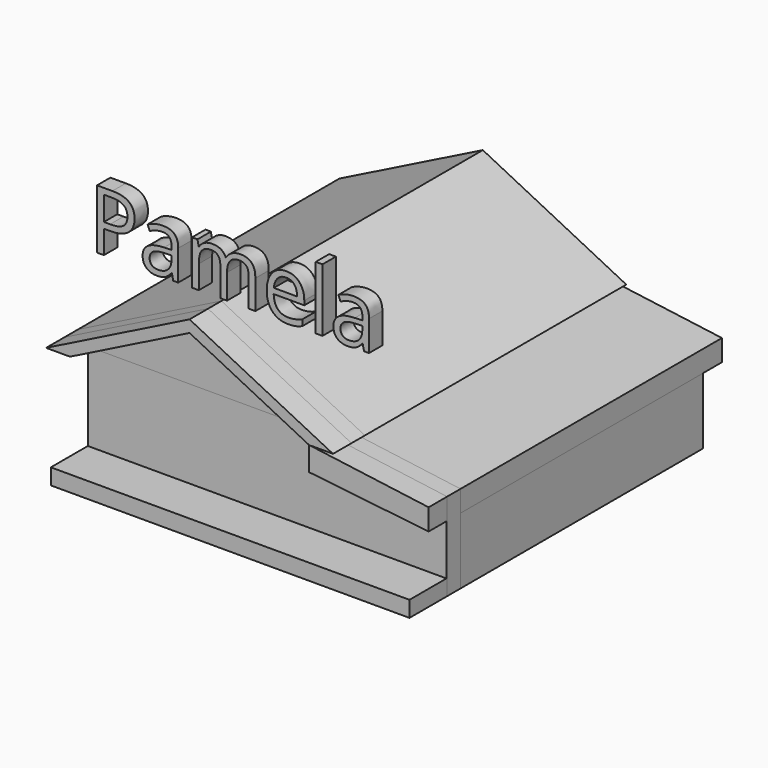
from build123d import *

# Parameters (mm, degrees)
F1_DEPTH      = 914.4
F1_DEPTH_BACK = 13106.4
F2_DEPTH      = 60.96
F2_DEPTH_BACK = 12192
F3_DEPTH      = 914.4
F3_DEPTH_BACK = 13106.4
F0_W          = 4572
F0_H          = 1371.6
F0_W_2        = 1219.2
F0_H_2        = 914.4
F0_W_3        = 4267.2
F0_H_3        = 1066.8
F0_W_4        = 914.4
F0_H_4        = 2133.6
F0_H_5        = 609.6
F4_DEPTH      = 60.96
F4_DEPTH_BACK = 12192
F6_DEPTH      = 1828.8
F6_DEPTH_BACK = 12192
F0_TEXT_SIZE  = 3172.1966134177
F7_DEPTH      = 30.48
F7_DEPTH_BACK = 609.6
F8_W          = 1219.2
F8_H          = 1524
F8_W_2        = 914.4
F8_H_2        = 1219.2
F9_DEPTH      = 152.4


# Not quite as in the source:
# - the program builds the solid bodies; features that only make, move or delete a surface that nothing else refers to are left out
# - Text() gives the source's letters only with a copy of the font that has no kerning and outlines rounded to 1/6400 em; it was checked with that copy


with BuildPart() as f1:
    # F0 (on Front) → F1 (new body, two sides)
    with BuildSketch(Plane.XZ) as f1_sk:
        Polygon((-5486.4, 0), (-4572, 0), (0, 2286), (0, 2743.2), align=None)
        Polygon((0, 2286), (4572, 0), (5486.4, 0), (0, 2743.2), align=None)
    extrude(amount=F1_DEPTH)
    extrude(f1_sk.sketch, amount=-F1_DEPTH_BACK)

    # F0 (on Front) → F2 (join, two sides)
    with BuildSketch(Plane.XZ) as f2_sk:
        Polygon((-4572, 0), (0, 0), (0, 2286), align=None)
        Polygon((0, 2286), (0, 0), (4572, 0), align=None)
    extrude(amount=F2_DEPTH)
    extrude(f2_sk.sketch, amount=-F2_DEPTH_BACK)


with BuildPart() as f3:
    # F0 (on Front) → F3 (new body, two sides)
    with BuildSketch(Plane.XZ) as f3_sk:
        Polygon((9144, -609.6), (4572, 0), (4572, -914.4), (9144, -1426.464), align=None)
    extrude(amount=F3_DEPTH)
    extrude(f3_sk.sketch, amount=-F3_DEPTH_BACK)


with BuildPart() as f4:
    # F0 (on Front) → F4 (new body, two sides)
    with BuildSketch(Plane.XZ) as f4_sk:
        Polygon((4572, 0), (0, 0), (-4572, 0), (-4572, -3352.8), (-3657.6, -3352.8), (-3657.6, -914.4), (-2133.6, -914.4), (-2133.6, -3352.8), (4572, -3352.8), (4572, -914.4), align=None)
        with Locations((1676.4, -1905)):
            Rectangle(F0_W, F0_H, mode=Mode.SUBTRACT)
        Polygon((9144, -1426.464), (4572, -914.4), (4572, -3352.8), (9144, -3352.8), align=None)
        with Locations((6400.8, -2133.6)):
            Rectangle(F0_W_2, F0_H_2, mode=Mode.SUBTRACT)
        with Locations((1676.4, -1905)):
            Rectangle(F0_W, F0_H)
        with Locations((1676.4, -1905)):
            Rectangle(F0_W_3, F0_H_3, mode=Mode.SUBTRACT)
        with Locations((1676.4, -1905)):
            Rectangle(F0_W_3, F0_H_3)
        with Locations((-2895.6, -2286)):
            Rectangle(F0_W_4, F0_H_4)
        Polygon((-3657.6, -914.4), (-3657.6, -3352.8), (-3352.8, -3352.8), (-3352.8, -1219.2), (-2438.4, -1219.2), (-2438.4, -3352.8), (-2133.6, -3352.8), (-2133.6, -914.4), align=None)
        with Locations((6400.8, -2133.6)):
            Rectangle(F0_W_2, F0_H_2)
        with Locations((6400.8, -2133.6)):
            Rectangle(F0_W_4, F0_H_5, mode=Mode.SUBTRACT)
        with Locations((6400.8, -2133.6)):
            Rectangle(F0_W_4, F0_H_5)
    extrude(amount=F4_DEPTH)
    extrude(f4_sk.sketch, amount=-F4_DEPTH_BACK)

    # F0 (on Front) → F6 (join, two sides)
    with BuildSketch(Plane.XZ) as f6_sk:
        Polygon((-3657.6, -3352.8), (-4572, -3352.8), (-4572, -3962.4), (4572, -3962.4), (4572, -3352.8), (-2133.6, -3352.8), (-2438.4, -3352.8), (-3352.8, -3352.8), align=None)
        with Locations((6858, -3657.6)):
            Rectangle(F0_W, F0_H_5)
    extrude(amount=F6_DEPTH)
    extrude(f6_sk.sketch, amount=-F6_DEPTH_BACK)

    # F8 (on face) → F9 (join)
    with BuildSketch(Plane(origin=(-4572, 0, 0), x_dir=(0, -1, 0), z_dir=(-1, 0, 0))):
        with Locations((-2346.96, -1402.08)):
            Rectangle(F8_W, F8_H)
        with Locations((-2346.96, -1402.08)):
            Rectangle(F8_W_2, F8_H_2, mode=Mode.SUBTRACT)
        with Locations((-9784.08, -1402.08)):
            Rectangle(F8_W, F8_H)
        with Locations((-9784.08, -1402.08)):
            Rectangle(F8_W_2, F8_H_2, mode=Mode.SUBTRACT)
    extrude(amount=F9_DEPTH)


with BuildPart() as f7:
    # F0 (on Front) → F7 (new body, two sides)
    with BuildSketch(Plane.XZ) as f7_sk:
        Polygon((4572, 0), (0, 0), (-4572, 0), (-4572, -3352.8), (-3657.6, -3352.8), (-3657.6, -914.4), (-2133.6, -914.4), (-2133.6, -3352.8), (4572, -3352.8), (4572, -914.4), align=None)
        with Locations((1676.4, -1905)):
            Rectangle(F0_W, F0_H, mode=Mode.SUBTRACT)
        Polygon((0, 2286), (0, 0), (4572, 0), align=None)
        Polygon((-4572, 0), (0, 0), (0, 2286), align=None)
        Polygon((-5486.4, 0), (-4572, 0), (0, 2286), (0, 2743.2), align=None)
        Polygon((0, 2286), (4572, 0), (5486.4, 0), (0, 2743.2), align=None)
        Polygon((9144, -609.6), (4572, 0), (4572, -914.4), (9144, -1426.464), align=None)
        Polygon((-3657.6, -3352.8), (-4572, -3352.8), (-4572, -3962.4), (4572, -3962.4), (4572, -3352.8), (-2133.6, -3352.8), (-2438.4, -3352.8), (-3352.8, -3352.8), align=None)
        Polygon((9144, -1426.464), (4572, -914.4), (4572, -3352.8), (9144, -3352.8), align=None)
        with Locations((6400.8, -2133.6)):
            Rectangle(F0_W_2, F0_H_2, mode=Mode.SUBTRACT)
        with Locations((6858, -3657.6)):
            Rectangle(F0_W, F0_H_5)
        with Locations((-4557.2702884674, 3250.6768703461)):
            Text('Pamela', F0_TEXT_SIZE, font='Open Sans', text_align=(TextAlign.LEFT, TextAlign.BOTTOM))
    extrude(amount=F7_DEPTH)
    extrude(f7_sk.sketch, amount=-F7_DEPTH_BACK)


solid = Compound([f1.part, f3.part, f4.part, f7.part])
